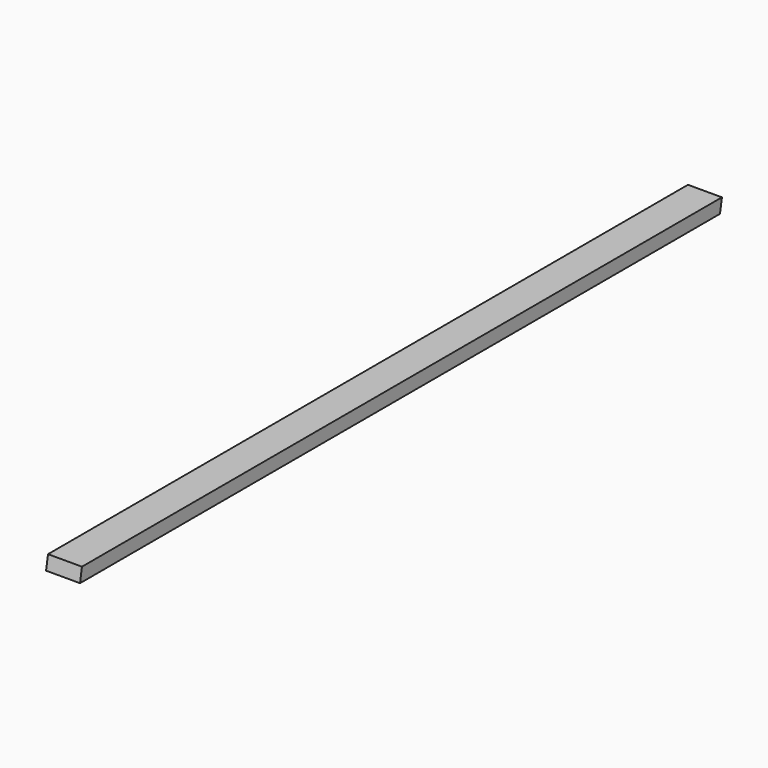
from build123d import *

# Parameters (mm, degrees)
F0_W     = 63.5
F0_H     = 1500.7336
F1_DEPTH = 25.4
F3_DEPTH = 63.501


# Not quite as in the source:
# - a feature names something its author has since deleted; it is built from what else it names


with BuildPart() as f1:
    # F0 (on Top) → F1 (new body)
    with BuildSketch(Plane.XY):
        with Locations((31.75, 750.3668)):
            Rectangle(F0_W, F0_H)
    extrude(amount=F1_DEPTH)

    # F2 (on face) → F3 (cut, through all)
    with BuildSketch(Plane.YZ.offset(63.5)):
        Polygon((0, 25.4), (0, 0), (4.47870531, 25.4), align=None)
        Polygon((1500.7336, 25.4), (1496.25489469, 0), (1500.7336, 0), align=None)
    extrude(amount=-F3_DEPTH, mode=Mode.SUBTRACT)


solid = f1.part
